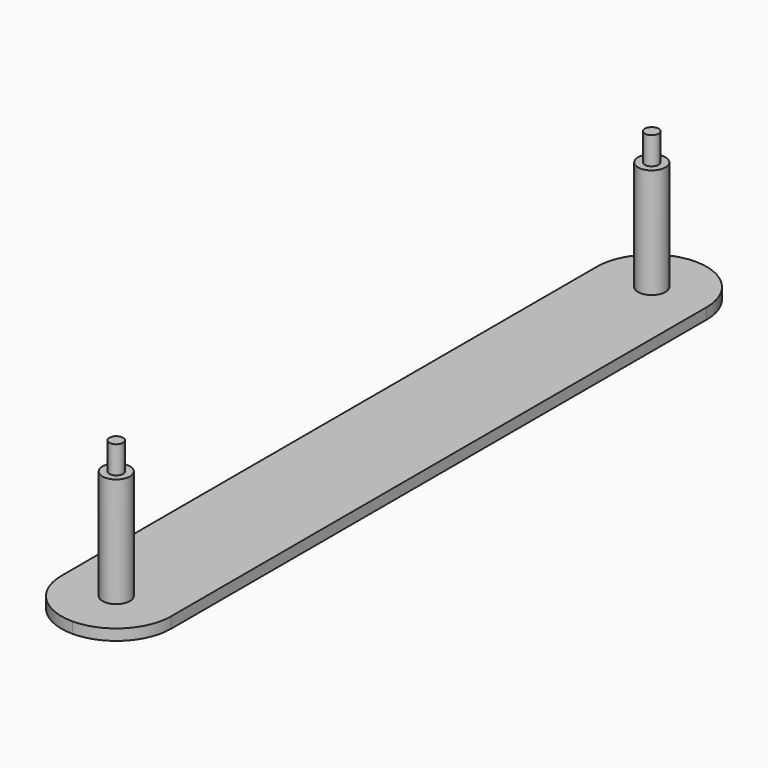
from build123d import *

# Parameters (mm, degrees)
F0_R     = 3.175
F0_R_2   = 1.5875
F1_DEPTH = 2.54
F2_DEPTH = 25.4
F3_R     = 12.69999
F4_DEPTH = 31.75


# Not quite as in the source:
# - a fillet or chamfer is up to 0.001 mm smaller than in the source, because OpenCascade refuses the exact size


with BuildPart() as f1:
    # F0 (on Top) → F1 (new body)
    with BuildSketch(Plane.XY):
        Polygon((12.7, 167.64), (0, 167.64), (-12.7, 167.64), (-12.7, -12.7), (0, -12.7), (12.7, -12.7), align=None)
        Circle(F0_R, mode=Mode.SUBTRACT)
        with Locations((0, 154.94)):
            Circle(F0_R, mode=Mode.SUBTRACT)
        with Locations((0, 154.94)):
            Circle(F0_R)
        with Locations((0, 154.94)):
            Circle(F0_R_2, mode=Mode.SUBTRACT)
        with Locations((0, 154.94)):
            Circle(F0_R_2)
        Circle(F0_R)
        Circle(F0_R_2, mode=Mode.SUBTRACT)
        Circle(F0_R_2)
    extrude(amount=-F1_DEPTH)

    # F0 (on Top) → F2 (join)
    with BuildSketch(Plane.XY):
        with Locations((0, 154.94)):
            Circle(F0_R)
        with Locations((0, 154.94)):
            Circle(F0_R_2, mode=Mode.SUBTRACT)
        Circle(F0_R)
        Circle(F0_R_2, mode=Mode.SUBTRACT)
        with Locations((0, 154.94)):
            Circle(F0_R_2)
        Circle(F0_R_2)
    extrude(amount=F2_DEPTH)

    # F3 (radius 12.7 in the source; OpenCascade refuses exactly that, so slightly less here)
    f3_edges = [f1.edges().sort_by_distance(p)[0] for p in [
        (12.7, 167.64, -1.27),
        (-12.7, 167.64, -1.27),
        (-12.7, -12.7, -1.27),
        (12.7, -12.7, -1.27),
    ]]
    fillet(f3_edges, radius=F3_R)

    # F0 (on Top) → F4 (join)
    with BuildSketch(Plane.XY):
        Circle(F0_R_2)
        with Locations((0, 154.94)):
            Circle(F0_R_2)
    extrude(amount=F4_DEPTH)


solid = f1.part
